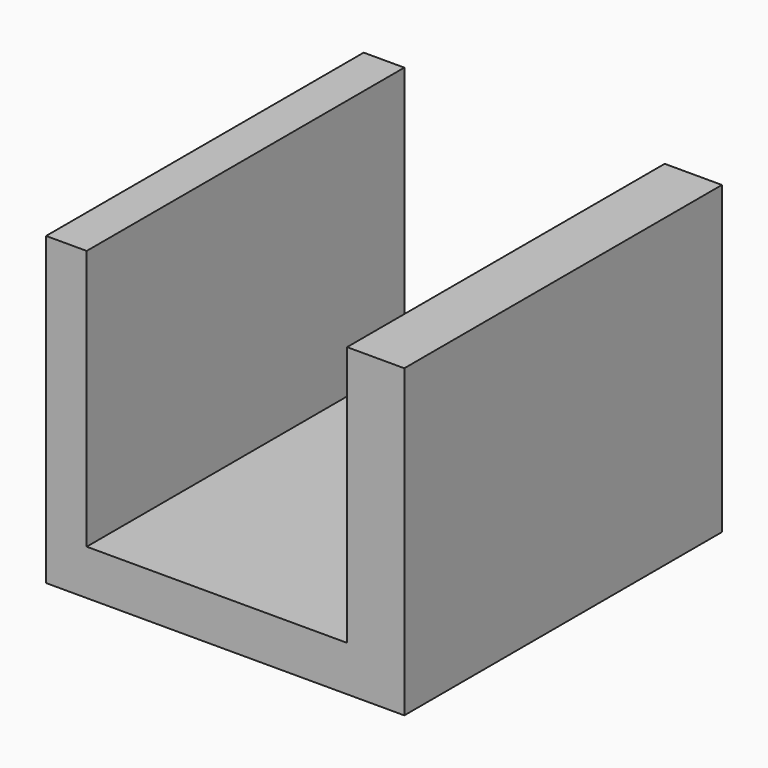
from build123d import *

# Parameters (mm, degrees)
F1_DEPTH = 65.532


# Not quite as in the source:
# - a feature names something its author has since deleted; it is built from what else it names


with BuildPart() as f1:
    # F0 (on Front) → F1 (new body)
    with BuildSketch(Plane.XZ):
        Polygon((-52.4255991913, 50.4443980753), (-59.1312013566, 50.4443980753), (-59.1312013566, 0), (0, 0), (0, 50.4443980753), (-9.4488011673, 50.4443980753), (-9.4488011673, 7.4676000513), (-52.4255991913, 7.4676000513), align=None)
    extrude(amount=F1_DEPTH)


solid = f1.part
